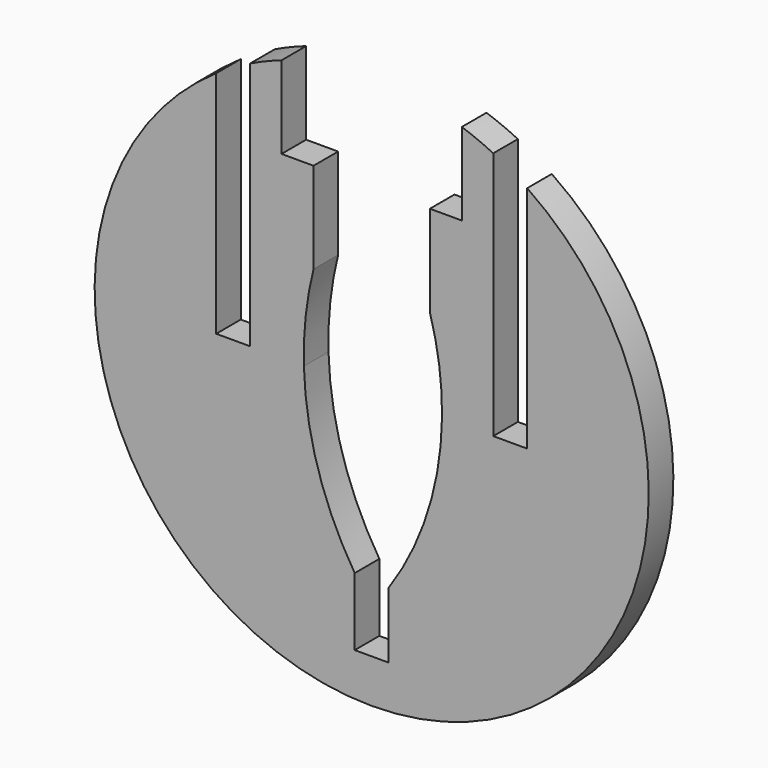
from build123d import *

# Parameters (mm, degrees)
F0_R     = 28.575
F1_DEPTH = 3.175
F3_DEPTH = 3.176


# Not quite as in the source:
# - a length typed as a fraction of an inch, garbled in the dataset ("3 / 203.2 mm" for 3/8 in), is restored


with BuildPart() as f1:
    # F0 (on Front) → F1 (new body)
    with BuildSketch(Plane.XZ):
        Circle(F0_R)
    extrude(amount=F1_DEPTH)

    # F2 (on face) → F3 (cut, through all)
    with BuildSketch(Plane.XZ.offset(3.175)):
        with BuildLine():
            Line((-1.75, -17.08304261), (-1.75, -24.075))
            Line((-1.75, -24.075), (0, -24.075))
            Line((0, -24.075), (0, -19.575))
            ThreePointArc((0, -19.575), (-0.9032383957, -18.3488519781), (-1.75, -17.08304261))
        make_face()
        with BuildLine():
            Line((0, -19.575), (0, -24.075))
            Line((0, -24.075), (1.75, -24.075))
            Line((1.75, -24.075), (1.75, -17.2770230976))
            ThreePointArc((1.75, -17.2770230976), (0.9017072988, -18.4463502097), (0, -19.575))
        make_face()
        with BuildLine():
            ThreePointArc((-6.9936556862, 0), (-5.528073584, -8.8964320017), (-1.75, -17.08304261))
            ThreePointArc((-1.75, -17.08304261), (-0.9032383957, -18.3488519781), (0, -19.575))
            Line((0, -19.575), (0, 0))
            Line((0, 0), (-6.9936556862, 0))
        make_face()
        with BuildLine():
            Line((0, 0), (0, -19.575))
            ThreePointArc((0, -19.575), (0.9017072988, -18.4463502097), (1.75, -17.2770230976))
            ThreePointArc((1.75, -17.2770230976), (5.789623043, -9.0487471984), (7.2536082684, 0))
            Line((7.2536082684, 0), (0, 0))
        make_face()
        with BuildLine():
            ThreePointArc((-6, 9.1323722154), (-6.8103344804, 4.6002974695), (-6.9936556862, 0))
            Line((-6.9936556862, 0), (0, 0))
            Line((0, 0), (7.2536082684, 0))
            ThreePointArc((7.2536082684, 0), (6.9672213091, 4.6129154541), (6, 9.1323722154))
            Line((6, 9.1323722154), (6, 18.5192639611))
            Line((6, 18.5192639611), (9.3, 18.5192639611))
            Line((9.3, 18.5192639611), (9.3, 27.0192639611))
            ThreePointArc((9.3, 27.0192639611), (0, 28.575), (-9.3, 27.0192639611))
            Line((-9.3, 27.0192639611), (-9.3, 18.5192639611))
            Line((-9.3, 18.5192639611), (-6, 18.5192639611))
            Line((-6, 18.5192639611), (-6, 9.1323722154))
        make_face()
        with BuildLine():
            Line((12.5375, 0), (16.0375, 0))
            Line((16.0375, 0), (16.0375, 23.650142045))
            ThreePointArc((16.0375, 23.650142045), (14.3234197578, 24.7259028438), (12.5375, 25.6776501797))
            Line((12.5375, 25.6776501797), (12.5375, 0))
        make_face()
        with BuildLine():
            Line((-16.0375, 0), (-12.5375, 0))
            Line((-12.5375, 0), (-12.5375, 25.6776501797))
            ThreePointArc((-12.5375, 25.6776501797), (-14.3234197578, 24.7259028438), (-16.0375, 23.650142045))
            Line((-16.0375, 23.650142045), (-16.0375, 0))
        make_face()
    extrude(amount=-F3_DEPTH, mode=Mode.SUBTRACT)


solid = f1.part
